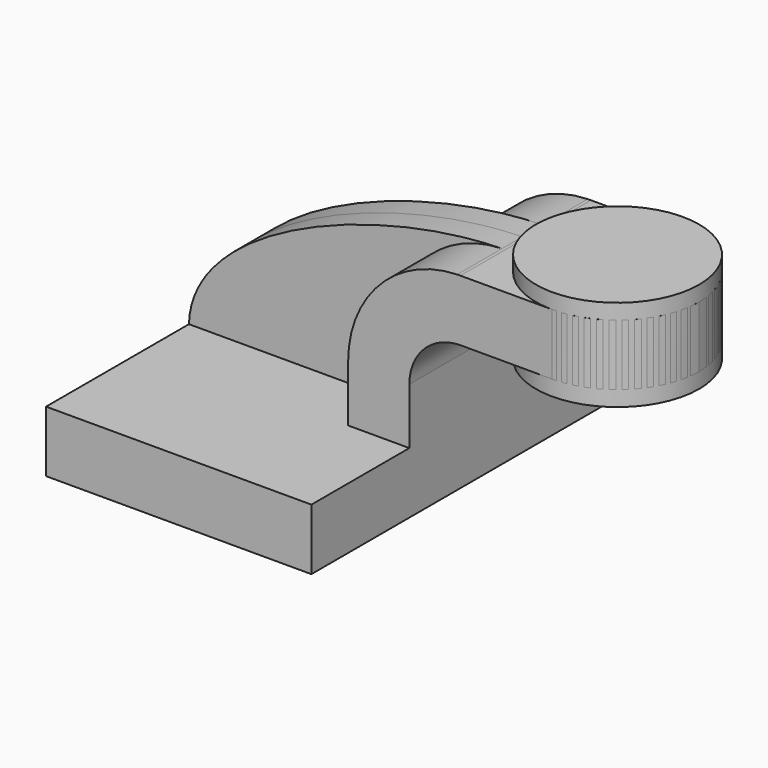
from build123d import *

# Parameters (mm, degrees)
F1_DEPTH = 63.5
F2_DEPTH = 25.4
F3_DEPTH = 7.9375
F4_DEPTH = 50.8
F6_R     = 25.39999


# Not quite as in the source:
# - a fillet or chamfer is up to 0.001 mm smaller than in the source, because OpenCascade refuses the exact size


with BuildPart() as f1:
    # F0 (on Front) → F1 (new body, symmetric)
    with BuildSketch(Plane.XZ):
        Polygon((-41.275, 9.525), (-41.275, -9.525), (41.275, -9.525), (41.275, 9.525), (22.225, 9.525), align=None)
    extrude(amount=F1_DEPTH, both=True)

    # F0 (on Front) → F2 (join, symmetric)
    with BuildSketch(Plane.XZ):
        with BuildLine():
            Line((22.225, 9.525), (41.275, 9.525))
            Line((41.275, 9.525), (41.275, 27.0002))
            ThreePointArc((41.275, 27.0002), (45.9246798487, 38.2255201513), (57.15, 42.8752))
            Line((57.15, 42.8752), (60.325, 42.8752))
            Line((60.325, 42.8752), (60.325, 61.9252))
            Line((60.325, 61.9252), (57.15, 61.9252))
            add(Edge.make_bspline(
                [(56.1497156539, 61.9108725261), (56.4844485329, 61.9171678859), (56.8178918504, 61.9219463376), (57.15, 61.9252)],
                knots=[110.5648551898, 110.5648551898, 110.5648551898, 110.5648551898, 111.5045361635, 111.5045361635, 111.5045361635, 111.5045361635], degree=3))
            ThreePointArc((56.1497156539, 61.9108725261), (32.1031383624, 51.3396812415), (22.225, 27.0002))
            Line((22.225, 27.0002), (22.225, 9.525))
        make_face()
    extrude(amount=F2_DEPTH, both=True)

    # F0 (on Front) → F3 (join, symmetric)
    with BuildSketch(Plane.XZ):
        with BuildLine():
            add(Edge.make_bspline(
                [(-41.275, 9.525), (-40.4742170634, 39.4287788878), (16.7643355785, 61.1701471538), (56.1497156539, 61.9108725261)],
                knots=[0, 0, 0, 0, 110.5648551898, 110.5648551898, 110.5648551898, 110.5648551898], degree=3))
            Line((-41.275, 9.525), (22.225, 9.525))
            Line((22.225, 9.525), (22.225, 27.0002))
            ThreePointArc((22.225, 27.0002), (32.1031383624, 51.3396812415), (56.1497156539, 61.9108725261))
        make_face()
    extrude(amount=F3_DEPTH, both=True)

    # F4 (add): a face of the model
    f4_faces = [f1.faces().sort_by_distance(p)[0] for p in [
        (60.325, 0, 52.4002),
    ]]
    extrude(f4_faces, amount=F4_DEPTH)

    # F6 (radius 25.4 in the source; OpenCascade refuses exactly that, so slightly less here)
    f6_edges = [f1.edges().sort_by_distance(p)[0] for p in [
        (111.125, -25.4, 52.4002),
        (111.125, 25.4, 52.4002),
    ]]
    fillet(f6_edges, radius=F6_R)


with BuildPart() as f5:
    # F0 (on Front) → F5 (revolve)
    with BuildSketch(Plane.XZ):
        Polygon((85.725, 66.675), (85.725, 61.9252), (85.725, 42.8752), (85.725, 38.1), (111.125, 38.1), (111.125, 66.675), align=None)
    revolve(axis=Axis((85.725, 0, 52.3875), (0, 0, 1)))


solid = Compound([f1.part, f5.part])
